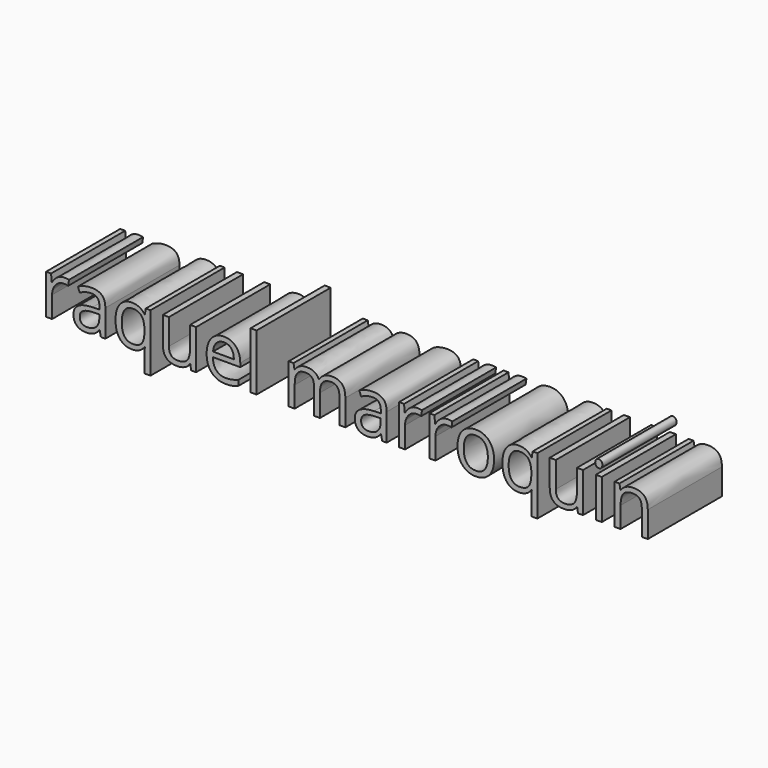
from build123d import *

# Parameters (mm, degrees)
F0_TEXT_SIZE = 8.0174080924
F1_DEPTH     = 10


# Not quite as in the source:
# - Text() gives the source's letters only with a copy of the font that has no kerning and outlines rounded to 1/6400 em; it was checked with that copy


with BuildPart() as f1:
    # F0 (on Front) → F1 (new body)
    with BuildSketch(Plane.XZ):
        with Locations((0, 0)):
            Text('raquel marroquin', F0_TEXT_SIZE, font='Open Sans', text_align=(TextAlign.LEFT, TextAlign.BOTTOM))
    extrude(amount=F1_DEPTH)


solid = f1.part
